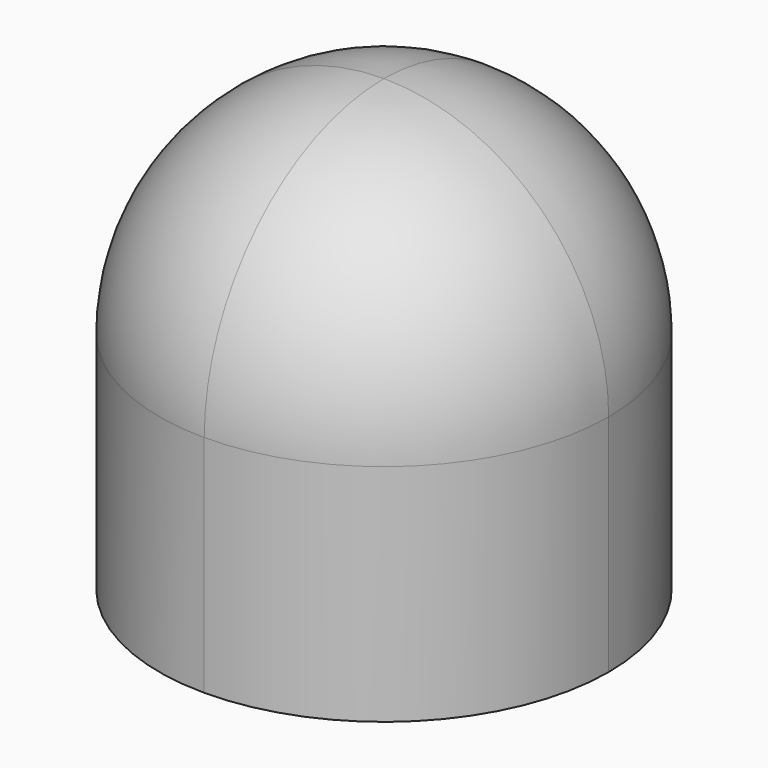
from build123d import *

# Parameters (mm, degrees)
F0_W     = 254
F0_H     = 254
F1_DEPTH = 254
F2_R     = 126.99999
F3_R     = 126.99999


# Not quite as in the source:
# - a fillet or chamfer is up to 0.001 mm smaller than in the source, because OpenCascade refuses the exact size


with BuildPart() as f1:
    # F0 (on Top) → F1 (new body)
    with BuildSketch(Plane.XY):
        with Locations((50.79993667, 50.8000484288)):
            Rectangle(F0_W, F0_H)
    extrude(amount=F1_DEPTH)

    # F2 (radius 127 in the source; OpenCascade refuses exactly that, so slightly less here)
    f2_edges = [f1.edges().sort_by_distance(p)[0] for p in [
        (-76.200063, 50.800048, 254),
        (177.799937, 50.800048, 254),
    ]]
    fillet(f2_edges, radius=F2_R)

    # F3 (radius 127 in the source; OpenCascade refuses exactly that, so slightly less here)
    f3_edges = [f1.edges().sort_by_distance(p)[0] for p in [
        (140.602501, 177.800048, 216.802564),
        (177.799937, 177.800048, 63.500005),
        (-76.200063, 177.800048, 63.500005),
        (140.602501, -76.199952, 216.802564),
    ]]
    fillet(f3_edges, radius=F3_R)


solid = f1.part
